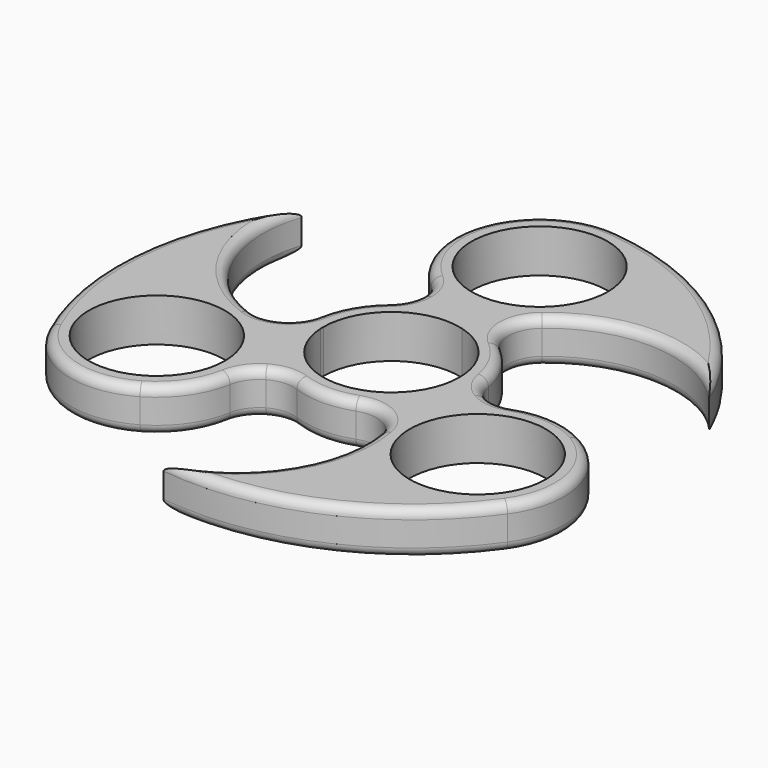
from build123d import *

# Parameters (mm, degrees)
F1_DEPTH = 7
F2_COUNT = 3
F3_R     = 1.5


# Not quite as in the source:
# - a feature names something its author has since deleted; it is built from what else it names


with BuildPart() as f1:
    # F0 (on Top) → F1 (new body)
    with BuildSketch(Plane.XY):
        with BuildLine():
            ThreePointArc((21.9951433725, -11.4925054907), (20.9459498097, -10.4148089852), (19.9779776986, -9.2636066213))
            ThreePointArc((19.9779776986, -9.2636066213), (8.7253710617, -9.681369457), (2.975, 0))
            Line((2.975, 0), (0, 0))
            ThreePointArc((0, 0), (7.5166369535, -12.4083038167), (21.9951433725, -11.4925054907))
        make_face()
        with BuildLine():
            ThreePointArc((2.975, 0), (7.3075898939, 8.7614081044), (16.9001287025, 10.6367231095))
            ThreePointArc((16.9001287025, 10.6367231095), (17.4750953036, 12.0265613368), (18.1496945041, 13.3708651748))
            ThreePointArc((18.1496945041, 13.3708651748), (11.2418636412, 13.7256214368), (5.0072992002, 10.7299269487))
            ThreePointArc((5.0072992002, 10.7299269487), (1.3134360208, 5.9203964733), (0, 0))
            Line((0, 0), (2.975, 0))
        make_face()
        with BuildLine():
            Line((25.025, 30), (28, 30))
            ThreePointArc((28, 30), (24.3806766846, 39.3936974387), (15.3940640614, 43.9304194263))
            ThreePointArc((15.3940640614, 43.9304194263), (4.6063025613, 40.3806766846), (0, 30))
            Line((0, 30), (2.975, 30))
            ThreePointArc((2.975, 30), (14, 41.025), (25.025, 30))
        make_face()
        with BuildLine():
            ThreePointArc((5.0072993058, 19.2700729627), (13.9999999193, 16), (22.9927005704, 19.270072859))
            ThreePointArc((22.9927005704, 19.270072859), (26.6865639159, 24.079603391), (28, 30))
            Line((28, 30), (25.025, 30))
            ThreePointArc((25.025, 30), (14, 18.975), (2.975, 30))
            Line((2.975, 30), (0, 30))
            ThreePointArc((0, 30), (1.3134360499, 24.0796034642), (5.0072993058, 19.2700729627))
        make_face()
        with BuildLine():
            ThreePointArc((16.9001287025, 10.6367231095), (22.7614081044, 6.6924101061), (25.025, 0))
            Line((25.025, 0), (28, 0))
            ThreePointArc((28, 0), (26.6865639463, 5.9203965438), (22.9927006805, 10.7299270487))
            ThreePointArc((22.9927006805, 10.7299270487), (20.702557448, 12.2912864931), (18.1496945041, 13.3708651748))
            ThreePointArc((18.1496945041, 13.3708651748), (17.4750953036, 12.0265613368), (16.9001287025, 10.6367231095))
        make_face()
        with BuildLine():
            ThreePointArc((18.1496945041, 13.3708651748), (20.702557448, 12.2912864931), (22.9927006805, 10.7299270487))
            ThreePointArc((22.9927006805, 10.7299270487), (21, 14.9999999282), (22.9927005704, 19.270072859))
            ThreePointArc((22.9927005704, 19.270072859), (20.2962936097, 16.5461537969), (18.1496945041, 13.3708651748))
        make_face()
        with BuildLine():
            Line((28, 0), (25.025, 0))
            ThreePointArc((25.025, 0), (23.681369457, -5.2746289383), (19.9779776986, -9.2636066213))
            ThreePointArc((19.9779776986, -9.2636066213), (20.9459498097, -10.4148089852), (21.9951433725, -11.4925054907))
            ThreePointArc((21.9951433725, -11.4925054907), (26.4083038167, -6.4833630465), (28, 0))
        make_face()
        with BuildLine():
            ThreePointArc((5.0072992002, 10.7299269487), (11.2418636412, 13.7256214368), (18.1496945041, 13.3708651748))
            ThreePointArc((18.1496945041, 13.3708651748), (20.2962936097, 16.5461537969), (22.9927005704, 19.270072859))
            ThreePointArc((22.9927005704, 19.270072859), (13.9999999193, 16), (5.0072993058, 19.2700729627))
            ThreePointArc((5.0072993058, 19.2700729627), (6.4773060756, 17.3560761428), (7, 15))
            ThreePointArc((7, 15), (6.4773060464, 12.6439237947), (5.0072992002, 10.7299269487))
        make_face()
        with BuildLine():
            ThreePointArc((28, 30), (26.6865639159, 24.079603391), (22.9927005704, 19.270072859))
            ThreePointArc((22.9927005704, 19.270072859), (37.7454683817, 24.0400706311), (51.6596345021, 17.1995284003))
            ThreePointArc((51.6596345021, 17.1995284003), (37.1930889334, 35.5389297837), (15.3940640614, 43.9304194263))
            ThreePointArc((15.3940640614, 43.9304194263), (24.3806766846, 39.3936974387), (28, 30))
        make_face()
    extrude(amount=F1_DEPTH)

    # F2: F1 ×3 about axis
    f2_axis = Axis((14, 0, 0), (0, 0, -1))


with BuildPart() as f1_1:
    add(f1.part)
    for i in range(1, F2_COUNT):
        add(f1.part.rotate(f2_axis, i * 360 / F2_COUNT))

    # F3
    f3_edges = [f1_1.edges().sort_by_distance(p)[0] for p in [
        (33.181072, -37.855269, 7),
        (22.946578, -32.584214, 7),
        (33.181072, -37.855269, 0),
        (37.193089, 35.53893, 7),
        (37.193089, 35.53893, 0),
        (22.946578, -32.584214, 0),
        (-28.37416, 2.316339, 0),
        (-10.235911, -28.890842, 0),
    ]]
    fillet(f3_edges, radius=F3_R)


solid = f1_1.part
